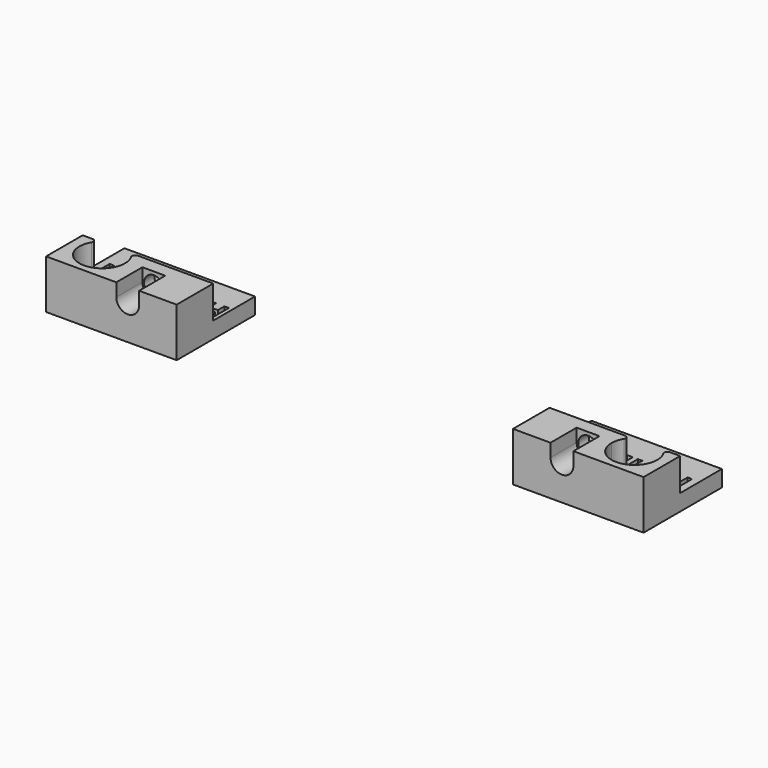
from build123d import *

# Parameters (mm, degrees)
F0_W      = 40
F0_H      = 30
F1_DEPTH  = 1
F3_DEPTH  = 4
F2_W      = 40
F2_H      = 16
F2_H_2    = 14
F2_W_2    = 2.5517578125
F2_H_3    = 2.7816840278
F4_DEPTH  = 4
F5_DEPTH  = 14
F6_R      = 3
F7_DEPTH  = 14
F9_DEPTH  = 10
F10_R     = 1
F11_DEPTH = 10


# Not quite as in the source:
# - a feature names something its author has since deleted; it is built from what else it names


with BuildPart() as f1:
    # F0 (on Top) → F1 (new body)
    with BuildSketch(Plane.XY):
        with Locations((-71.5087300752, 25.3250645474)):
            Rectangle(F0_W, F0_H)
    extrude(amount=F1_DEPTH)

    # F2 (on face) → F3 (join)
    with BuildSketch(Plane.XY.offset(1)):
        with BuildLine():
            Line((-61.5005737063, 31.8250645474), (-90.0087300752, 31.8250645474))
            Line((-90.0087300752, 31.8250645474), (-90.0087300752, 25.3250645474))
            Line((-90.0087300752, 25.3250645474), (-89.1976406655, 25.3250645474))
            Line((-89.1976406655, 25.3250645474), (-89.1976406655, 31.7700515265))
            Line((-89.1976406655, 31.7700515265), (-87.8307786863, 31.7700515265))
            Line((-87.8307786863, 31.7700515265), (-87.8307786863, 26.4535367696))
            Line((-87.8307786863, 26.4535367696), (-85.2169549016, 26.4535367696))
            Line((-85.2169549016, 26.4535367696), (-85.2169549016, 25.3250645474))
            Line((-85.2169549016, 25.3250645474), (-84.9080356308, 25.3250645474))
            Line((-84.9080356308, 25.3250645474), (-82.6327535127, 31.7968527418))
            Line((-82.6327535127, 31.7968527418), (-80.9626146238, 31.7968527418))
            Line((-80.9626146238, 31.7968527418), (-78.6788689641, 25.3250645474))
            Line((-78.6788689641, 25.3250645474), (-76.1440009832, 25.3250645474))
            add(Edge.make_bspline(
                [(-76.1440009832, 25.3250645474), (-76.7929122983, 25.4742321182), (-77.2238450926, 25.8737841654)],
                knots=[0.3733370206, 0.3733370206, 0.3733370206, 1, 1, 1], degree=2))
            add(Edge.make_bspline(
                [(-77.2238450926, 25.8737841654), (-77.911507853, 26.511370971), (-77.911507853, 27.6172737487)],
                knots=[0, 0, 0, 1, 1, 1], degree=2))
            Line((-77.911507853, 27.6172737487), (-77.911507853, 31.7700515265))
            Line((-77.911507853, 31.7700515265), (-76.5502882349, 31.7700515265))
            Line((-76.5502882349, 31.7700515265), (-76.5502882349, 27.8246305196))
            add(Edge.make_bspline(
                [(-76.5502882349, 27.8246305196), (-76.5502882349, 27.0798388529), (-76.2505378009, 26.7314230543)],
                knots=[0, 0, 0, 1, 1, 1], degree=2))
            add(Edge.make_bspline(
                [(-76.2505378009, 26.7314230543), (-75.9507873669, 26.3830072557), (-75.2581875405, 26.3830072557)],
                knots=[0, 0, 0, 1, 1, 1], degree=2))
            add(Edge.make_bspline(
                [(-75.2581875405, 26.3830072557), (-74.5881571585, 26.3830072557), (-74.2862908391, 26.7335389397)],
                knots=[0, 0, 0, 1, 1, 1], degree=2))
            add(Edge.make_bspline(
                [(-74.2862908391, 26.7335389397), (-73.9844245196, 27.0840706237), (-73.9844245196, 27.8330940612)],
                knots=[0, 0, 0, 1, 1, 1], degree=2))
            Line((-73.9844245196, 27.8330940612), (-73.9844245196, 31.7700515265))
            Line((-73.9844245196, 31.7700515265), (-72.6217943113, 31.7700515265))
            Line((-72.6217943113, 31.7700515265), (-72.6217943113, 27.6003466654))
            add(Edge.make_bspline(
                [(-72.6217943113, 27.6003466654), (-72.6217943113, 26.8851773946), (-72.9412930092, 26.3477424987)],
                knots=[0, 0, 0, 1, 1, 1], degree=2))
            add(Edge.make_bspline(
                [(-72.9412930092, 26.3477424987), (-73.2607917071, 25.8103076029), (-73.8652296412, 25.5232524814)],
                knots=[0, 0, 0, 1, 1, 1], degree=2))
            add(Edge.make_bspline(
                [(-73.8652296412, 25.5232524814), (-74.1333575757, 25.3959151776), (-74.4446485457, 25.3250645474)],
                knots=[0, 0, 0, 0.4435987872, 0.4435987872, 0.4435987872], degree=2))
            Line((-74.4446485457, 25.3250645474), (-71.0433437905, 25.3250645474))
            Line((-71.0433437905, 25.3250645474), (-71.0433437905, 31.7700515265))
            Line((-71.0433437905, 31.7700515265), (-69.319602471, 31.7700515265))
            Line((-69.319602471, 31.7700515265), (-66.5209913599, 26.943011596))
            Line((-66.5209913599, 26.943011596), (-66.4899583738, 26.943011596))
            add(Edge.make_bspline(
                [(-66.4899583738, 26.943011596), (-66.5562561169, 28.1998475335), (-66.5562561169, 28.7189447557)],
                knots=[0, 0, 0, 1, 1, 1], degree=2))
            Line((-66.5562561169, 28.7189447557), (-66.5562561169, 31.7700515265))
            Line((-66.5562561169, 31.7700515265), (-65.3262213946, 31.7700515265))
            Line((-65.3262213946, 31.7700515265), (-65.3262213946, 25.3250645474))
            Line((-65.3262213946, 25.3250645474), (-61.9332105806, 25.3250645474))
            add(Edge.make_bspline(
                [(-61.9332105806, 25.3250645474), (-62.7411498094, 25.5115877925), (-63.2456007349, 26.0896044779)],
                knots=[0.3226952609, 0.3226952609, 0.3226952609, 1, 1, 1], degree=2))
            add(Edge.make_bspline(
                [(-63.2456007349, 26.0896044779), (-63.9903924016, 26.943011596), (-63.9903924016, 28.5383892001)],
                knots=[0, 0, 0, 1, 1, 1], degree=2))
            add(Edge.make_bspline(
                [(-63.9903924016, 28.5383892001), (-63.9903924016, 29.5441400682), (-63.6243442245, 30.3002164571)],
                knots=[0, 0, 0, 1, 1, 1], degree=2))
            add(Edge.make_bspline(
                [(-63.6243442245, 30.3002164571), (-63.2582960474, 31.056292846), (-62.5727491724, 31.4590163703)],
                knots=[0, 0, 0, 1, 1, 1], degree=2))
            add(Edge.make_bspline(
                [(-62.5727491724, 31.4590163703), (-62.0940833767, 31.7402079025), (-61.5005737063, 31.8250645474)],
                knots=[0, 0, 0, 0.6982247505, 0.6982247505, 0.6982247505], degree=2))
        make_face()
        with BuildLine():
            Line((-52.0850104571, 31.8250645474), (-60.4313541686, 31.8250645474))
            add(Edge.make_bspline(
                [(-60.4313541686, 31.8250645474), (-59.7582676864, 31.7328733818), (-59.0801276446, 31.4089404154)],
                knots=[0.2845995164, 0.2845995164, 0.2845995164, 1, 1, 1], degree=2))
            Line((-59.0801276446, 31.4089404154), (-59.5202318113, 30.2973952765))
            add(Edge.make_bspline(
                [(-59.5202318113, 30.2973952765), (-59.8827535127, 30.4694872904), (-60.2480963946, 30.5971457106)],
                knots=[0, 0, 0, 1, 1, 1], degree=2))
            add(Edge.make_bspline(
                [(-60.2480963946, 30.5971457106), (-60.6134392766, 30.7248041307), (-60.966086846, 30.7248041307)],
                knots=[0, 0, 0, 1, 1, 1], degree=2))
            add(Edge.make_bspline(
                [(-60.966086846, 30.7248041307), (-61.737679728, 30.7248041307), (-62.1608568113, 30.1450515265)],
                knots=[0, 0, 0, 1, 1, 1], degree=2))
            add(Edge.make_bspline(
                [(-62.1608568113, 30.1450515265), (-62.5840338946, 29.5652989224), (-62.5840338946, 28.5299256585)],
                knots=[0, 0, 0, 1, 1, 1], degree=2))
            add(Edge.make_bspline(
                [(-62.5840338946, 28.5299256585), (-62.5840338946, 26.374543714), (-60.966086846, 26.374543714)],
                knots=[0, 0, 0, 1, 1, 1], degree=2))
            add(Edge.make_bspline(
                [(-60.966086846, 26.374543714), (-60.2875929224, 26.374543714), (-59.3227491724, 26.7130853807)],
                knots=[0, 0, 0, 1, 1, 1], degree=2))
            Line((-59.3227491724, 26.7130853807), (-59.3227491724, 25.5676860751))
            add(Edge.make_bspline(
                [(-59.3227491724, 25.5676860751), (-59.7050383524, 25.4078320586), (-60.1306271864, 25.3250645474)],
                knots=[0, 0, 0, 0.4822306436, 0.4822306436, 0.4822306436], degree=2))
            Line((-60.1306271864, 25.3250645474), (-57.9516554224, 25.3250645474))
            Line((-57.9516554224, 25.3250645474), (-57.9516554224, 31.7700515265))
            Line((-57.9516554224, 31.7700515265), (-56.5847934433, 31.7700515265))
            Line((-56.5847934433, 31.7700515265), (-56.5847934433, 29.243684339))
            Line((-56.5847934433, 29.243684339), (-54.0330356308, 29.243684339))
            Line((-54.0330356308, 29.243684339), (-54.0330356308, 31.7700515265))
            Line((-54.0330356308, 31.7700515265), (-52.6704054224, 31.7700515265))
            Line((-52.6704054224, 31.7700515265), (-52.6704054224, 25.3250645474))
            Line((-52.6704054224, 25.3250645474), (-52.0850104571, 25.3250645474))
            Line((-52.0850104571, 25.3250645474), (-52.0850104571, 31.8250645474))
        make_face()
    extrude(amount=F3_DEPTH)

    # F2 (on face) → F4 (join)
    with BuildSketch(Plane.XY.offset(1)):
        with Locations((-71.5087300752, 32.3250645474)):
            Rectangle(F2_W, F2_H)
        with BuildLine():
            Line((-90.0087300752, 25.3250645474), (-90.0087300752, 31.8250645474))
            Line((-90.0087300752, 31.8250645474), (-61.5005737063, 31.8250645474))
            add(Edge.make_bspline(
                [(-61.5005737063, 31.8250645474), (-61.2440566912, 31.8617398946), (-60.966086846, 31.8617398946)],
                knots=[0.6982247505, 0.6982247505, 0.6982247505, 1, 1, 1], degree=2))
            add(Edge.make_bspline(
                [(-60.966086846, 31.8617398946), (-60.6991203943, 31.8617398946), (-60.4313541686, 31.8250645474)],
                knots=[0, 0, 0, 0.2845995164, 0.2845995164, 0.2845995164], degree=2))
            Line((-60.4313541686, 31.8250645474), (-52.0850104571, 31.8250645474))
            Line((-52.0850104571, 31.8250645474), (-52.0850104571, 25.3250645474))
            Line((-52.0850104571, 25.3250645474), (-52.6704054224, 25.3250645474))
            Line((-52.6704054224, 25.3250645474), (-54.0330356308, 25.3250645474))
            Line((-54.0330356308, 25.3250645474), (-56.5847934433, 25.3250645474))
            Line((-56.5847934433, 25.3250645474), (-57.9516554224, 25.3250645474))
            Line((-57.9516554224, 25.3250645474), (-60.1306271864, 25.3250645474))
            add(Edge.make_bspline(
                [(-60.1306271864, 25.3250645474), (-60.5875804297, 25.2361973599), (-61.0944505613, 25.2361973599)],
                knots=[0.4822306436, 0.4822306436, 0.4822306436, 1, 1, 1], degree=2))
            add(Edge.make_bspline(
                [(-61.0944505613, 25.2361973599), (-61.5482757866, 25.2361973599), (-61.9332105806, 25.3250645474)],
                knots=[0, 0, 0, 0.3226952609, 0.3226952609, 0.3226952609], degree=2))
            Line((-61.9332105806, 25.3250645474), (-65.3262213946, 25.3250645474))
            Line((-65.3262213946, 25.3250645474), (-67.0626580266, 25.3250645474))
            Line((-67.0626580266, 25.3250645474), (-69.8217726099, 25.3250645474))
            Line((-69.8217726099, 25.3250645474), (-71.0433437905, 25.3250645474))
            Line((-71.0433437905, 25.3250645474), (-74.4446485457, 25.3250645474))
            add(Edge.make_bspline(
                [(-74.4446485457, 25.3250645474), (-74.8350974789, 25.2361973599), (-75.2934522974, 25.2361973599)],
                knots=[0.4435987872, 0.4435987872, 0.4435987872, 1, 1, 1], degree=2))
            add(Edge.make_bspline(
                [(-75.2934522974, 25.2361973599), (-75.757409426, 25.2361973599), (-76.1440009832, 25.3250645474)],
                knots=[0, 0, 0, 0.3733370206, 0.3733370206, 0.3733370206], degree=2))
            Line((-76.1440009832, 25.3250645474), (-78.6788689641, 25.3250645474))
            Line((-78.6788689641, 25.3250645474), (-80.1515252141, 25.3250645474))
            Line((-80.1515252141, 25.3250645474), (-83.4353793808, 25.3250645474))
            Line((-83.4353793808, 25.3250645474), (-84.9080356308, 25.3250645474))
            Line((-84.9080356308, 25.3250645474), (-85.2169549016, 25.3250645474))
            Line((-85.2169549016, 25.3250645474), (-89.1976406655, 25.3250645474))
            Line((-89.1976406655, 25.3250645474), (-90.0087300752, 25.3250645474))
        make_face(mode=Mode.SUBTRACT)
        with Locations((-71.5087300752, 17.3250645474)):
            Rectangle(F2_W, F2_H_2)
        with Locations((-55.308914537, 26.7159065612)):
            Rectangle(F2_W_2, F2_H_3)
        with BuildLine():
            Line((-82.624289971, 28.0051860751), (-80.9456875405, 28.0051860751))
            add(Edge.make_bspline(
                [(-80.9456875405, 28.0051860751), (-81.593148478, 30.0900385057), (-81.6749627141, 30.3636930196)],
                knots=[0, 0, 0, 1, 1, 1], degree=2))
            add(Edge.make_bspline(
                [(-81.6749627141, 30.3636930196), (-81.7567769502, 30.6373475335), (-81.7920417071, 30.7953336446)],
                knots=[0, 0, 0, 1, 1, 1], degree=2))
            add(Edge.make_bspline(
                [(-81.7920417071, 30.7953336446), (-81.9373325058, 30.2310975335), (-82.624289971, 28.0051860751)],
                knots=[0, 0, 0, 1, 1, 1], degree=2))
        make_face()
        Polygon((-82.9684739988, 26.8597867696), (-83.4353793808, 25.3250645474), (-80.1515252141, 25.3250645474), (-80.618430596, 26.8597867696), align=None)
        with BuildLine():
            Line((-69.8217726099, 25.3250645474), (-67.0626580266, 25.3250645474))
            Line((-67.0626580266, 25.3250645474), (-69.8669114988, 30.2000645474))
            Line((-69.8669114988, 30.2000645474), (-69.9064080266, 30.2000645474))
            add(Edge.make_bspline(
                [(-69.9064080266, 30.2000645474), (-69.8217726099, 28.9093744432), (-69.8217726099, 28.3578336446)],
                knots=[0, 0, 0, 1, 1, 1], degree=2))
            Line((-69.8217726099, 28.3578336446), (-69.8217726099, 25.3250645474))
        make_face()
    extrude(amount=F4_DEPTH)

    # F2 (on face) → F5 (join)
    with BuildSketch(Plane.XY.offset(1)):
        with Locations((-71.5087300752, 17.3250645474)):
            Rectangle(F2_W, F2_H_2)
    extrude(amount=F5_DEPTH)

    # F6 (on face) → F7 (cut)
    with BuildSketch(Plane.XZ.offset(-10.3250645474)):
        with Locations((-66.5087300752, 11)):
            Circle(F6_R)
    extrude(amount=-F7_DEPTH, mode=Mode.SUBTRACT)

    # F8 (on face) → F9 (cut)
    with BuildSketch(Plane.XY.offset(15)):
        with BuildLine():
            ThreePointArc((-86.4077095608, 24.3250645474), (-84.2204770768, 12.871660159), (-74.5087300752, 19.3250645474))
            ThreePointArc((-74.5087300752, 19.3250645474), (-75.0553256869, 22.0368115489), (-76.6097505896, 24.3250645474))
            Line((-76.6097505896, 24.3250645474), (-86.4077095608, 24.3250645474))
        make_face()
    extrude(amount=-F9_DEPTH, mode=Mode.SUBTRACT)

    # F10
    f10_edges = [f1.edges().sort_by_distance(p)[0] for p in [
        (-76.609751, 24.325065, 10),
        (-86.40771, 24.325065, 10),
    ]]
    fillet(f10_edges, radius=F10_R)

    # F6 (on face) → F11 (cut)
    with BuildSketch(Plane.XZ.offset(-10.3250645474)):
        with BuildLine():
            Line((-70.0087300752, 15), (-70.0087300752, 11))
            ThreePointArc((-70.0087300752, 11), (-66.5087300752, 7.5), (-63.0087300752, 11))
            Line((-63.0087300752, 11), (-63.0087300752, 15))
            Line((-63.0087300752, 15), (-70.0087300752, 15))
        make_face()
        with Locations((-66.5087300752, 11)):
            Circle(F6_R, mode=Mode.SUBTRACT)
    extrude(amount=-F11_DEPTH, mode=Mode.SUBTRACT)


with BuildPart() as f12_1:
    # F12: instance of F1
    add(f1.part.mirror(Plane.YZ))


solid = Compound([f1.part, f12_1.part])
